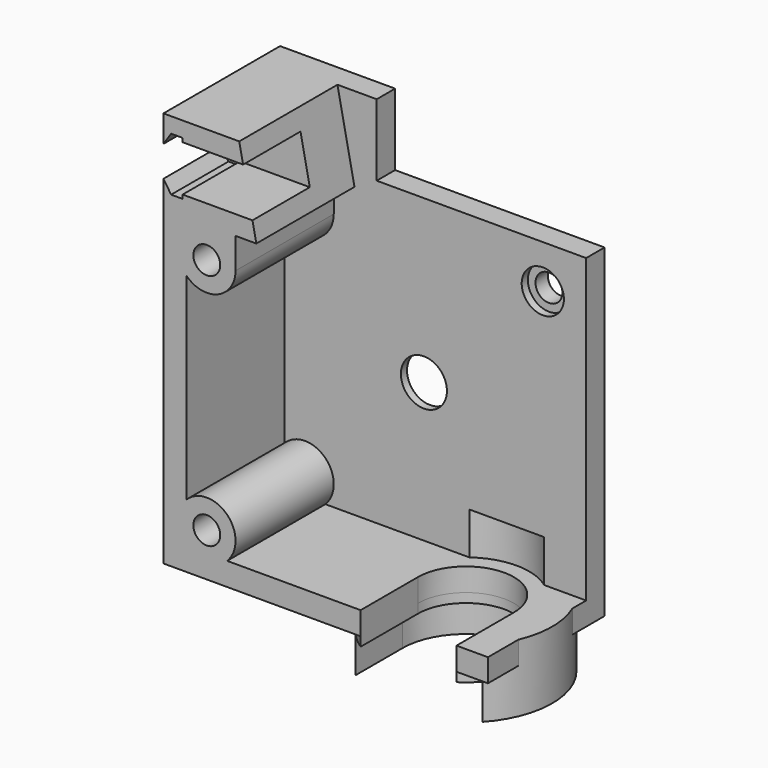
from build123d import *

# Parameters (mm, degrees)
F0_W      = 42.3
F0_H      = 42.3
F0_R      = 1.75
F0_R_2    = 3
F1_DEPTH  = 3
F2_R      = 11.5
F3_DEPTH  = 2
F4_R      = 1.75
F5_DEPTH  = 16
F9_W      = 15
F9_H      = 11
F10_DEPTH = 19
F11_DEPTH = 10
F18_DEPTH = 11.251
F19_W     = 28.3221583813
F19_H     = 99.7033566236
F20_DEPTH = 22.051
F22_DEPTH = 16.0051434669
F23_R     = 2.75
F23_R_2   = 1.75
F24_DEPTH = 1


# Not quite as in the source:
# - a feature names something its author has since deleted; it is built from what else it names


with BuildPart() as f1:
    # F0 (on Front) → F1 (new body)
    with BuildSketch(Plane.XZ):
        Rectangle(F0_W, F0_H)
        with Locations((-15.5, -15.5)):
            Circle(F0_R, mode=Mode.SUBTRACT)
        with Locations((-15.5, 15.5)):
            Circle(F0_R, mode=Mode.SUBTRACT)
        Circle(F0_R_2, mode=Mode.SUBTRACT)
        with Locations((15.5, 15.5)):
            Circle(F0_R, mode=Mode.SUBTRACT)
    extrude(amount=F1_DEPTH)

    # F2 (on face) → F3 (cut)
    with BuildSketch(Plane(origin=(0, 0, 0), x_dir=(-1, 0, 0), z_dir=(0, 1, 0))):
        Circle(F2_R)
    extrude(amount=-F3_DEPTH, mode=Mode.SUBTRACT)

    # F4 (on face) → F5 (join)
    with BuildSketch(Plane.XZ.offset(3)):
        with BuildLine():
            Line((-11.75, 21.15), (-21.15, 21.15))
            Line((-21.15, 21.15), (-21.15, -21.15))
            Line((-21.15, -21.15), (21.15, -21.15))
            Line((21.15, -21.15), (21.15, -18.15))
            Line((21.15, -18.15), (-12.8467001677, -18.15))
            ThreePointArc((-12.8467001677, -18.15), (-12.8483495706, -12.8483495706), (-18.15, -12.8467001677))
            Line((-18.15, -12.8467001677), (-18.15, 12.8467001677))
            ThreePointArc((-18.15, 12.8467001677), (-14.0638593384, 12.0358983849), (-11.75, 15.5))
            Line((-11.75, 15.5), (-11.75, 21.15))
        make_face()
        with Locations((-15.5, -15.5)):
            Circle(F4_R, mode=Mode.SUBTRACT)
        with Locations((-15.5, 15.5)):
            Circle(F4_R, mode=Mode.SUBTRACT)
    extrude(amount=F5_DEPTH)

    # F9 (on Front) → F10 (join, through all)
    with BuildSketch(Plane.XZ):
        with Locations((-13.65, 25)):
            Rectangle(F9_W, F9_H)
    extrude(amount=F10_DEPTH)

    # F8 (on offset) → F11 (cut)
    with BuildSketch(Plane.XZ.offset(9.65)):
        Polygon((0, 22), (0, 28), (-18.65, 28), (-18.65, 28.5), (-20.15, 28.5), (-21.15, 27), (-21.15, 23), (-20.15, 21.5), (-18.65, 21.5), (-18.65, 22), align=None)
    extrude(amount=F11_DEPTH, mode=Mode.SUBTRACT)

    # F13 (on offset) → F14 (revolve, cut)
    with BuildSketch(Plane.XZ.offset(9.65)):
        Polygon((17.05, -18.15), (19.05, -18.15), (19.05, -12.65), (10.8, -12.65), (10.8, -26.95), (19.05, -26.95), (19.05, -22.35), (17.05, -22.35), align=None)
    revolve(axis=Axis((10.8, -9.65, -5.160998553), (0, 0, -1)), mode=Mode.SUBTRACT)

    # F15 (on offset) → F16 (revolve)
    with BuildSketch(Plane.XZ.offset(9.65)):
        Polygon((19.05, -18.15), (17.05, -18.15), (17.05, -22.35), (19.05, -22.35), (19.05, -26.95), (22.05, -26.95), (22.05, -18.15), align=None)
    revolve(axis=Axis((10.8, -9.65, -5.160998553), (0, 0, -1)))

    # F17 (on offset) → F18 (cut, through all)
    with BuildSketch(Plane.XZ.offset(9.65)):
        Polygon((2.55, -12.65), (2.55, -18.15), (4.55, -18.15), (4.55, -22.35), (2.55, -22.35), (2.55, -26.95), (19.05, -26.95), (19.05, -22.35), (17.05, -22.35), (17.05, -18.15), (19.05, -18.15), (19.05, -12.65), align=None)
    extrude(amount=F18_DEPTH, mode=Mode.SUBTRACT)

    # F19 (on Right) → F20 (cut, through all)
    with BuildSketch(Plane.YZ):
        with Locations((14.1610791907, -2.7998201549)):
            Rectangle(F19_W, F19_H)
    extrude(amount=F20_DEPTH, mode=Mode.SUBTRACT)

    # F21 (on face) → F22 (cut, through all)
    with BuildSketch(Plane.XZ.offset(3)):
        with BuildLine():
            ThreePointArc((-4.9008020267, -0.9910295129), (0.9910295129, -4.9008020267), (4.9008020267, 0.9910295129))
            Line((4.9008020267, 0.9910295129), (-4.0184635896, 45.0982477529))
            ThreePointArc((-4.0184635896, 45.0982477529), (-9.9102951291, 49.0080202666), (-13.8200676429, 43.116188727))
            Line((-13.8200676429, 43.116188727), (-4.9008020267, -0.9910295129))
        make_face()
    extrude(amount=F22_DEPTH, mode=Mode.SUBTRACT)

    # F23 (on face) → F24 (cut)
    with BuildSketch(Plane.XZ.offset(3)):
        with Locations((15.5, 15.5)):
            Circle(F23_R)
        with Locations((15.5, 15.5)):
            Circle(F23_R_2, mode=Mode.SUBTRACT)
    extrude(amount=-F24_DEPTH, mode=Mode.SUBTRACT)


solid = f1.part
